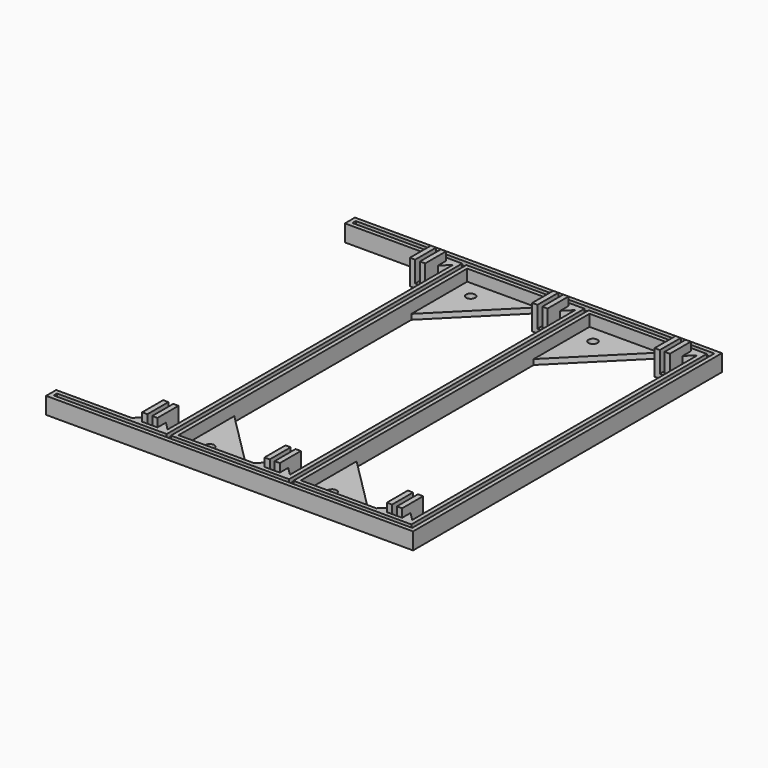
from build123d import *

# Parameters (mm, degrees)
F1_DEPTH     = 8
F2_W         = 2.5
F2_H         = 12.5
F3_DEPTH     = 4
F4_W         = 7.3
F4_H         = 12.5
F5_DEPTH     = 2
F7_DEPTH     = 2
F9_DEPTH     = 2
F10_T1_DEPTH = 8
F11_R        = 2.15
F12_DEPTH    = 2.5


# Not quite as in the source:
# - a fillet or chamfer that OpenCascade refuses, or shapes differently, is made with other operations: its cross-section is extruded or revolved along the edge and cut away or added


with BuildPart() as f1:
    # F0 (on Top) → F1 (new body)
    with BuildSketch(Plane.XY):
        Polygon((87.45, 92), (-87.45, 92), (-87.45, 86), (-46.45, 86), (-46.45, 73.5), (-43.95, 73.5), (-43.95, 86), (-41.65, 86), (-41.65, 73.5), (-39.15, 73.5), (-39.15, 86), (-35.15, 86), (-35.15, 0), (-35.15, -86), (-39.15, -86), (-39.15, -73.5), (-41.65, -73.5), (-41.65, -86), (-43.95, -86), (-43.95, -73.5), (-46.45, -73.5), (-46.45, -86), (-87.45, -86), (-87.45, -92), (87.45, -92), (87.45, 0), align=None)
        Polygon((-29.15, -86), (-29.15, 0), (-29.15, 86), (11.85, 86), (11.85, 73.5), (14.35, 73.5), (14.35, 86), (16.65, 86), (16.65, 73.5), (19.15, 73.5), (19.15, 86), (23.15, 86), (23.15, 0), (23.15, -86), (19.15, -86), (19.15, -73.5), (16.65, -73.5), (16.65, -86), (14.35, -86), (14.35, -73.5), (11.85, -73.5), (11.85, -86), align=None, mode=Mode.SUBTRACT)
        Polygon((29.15, -86), (29.15, 0), (29.15, 86), (70.15, 86), (70.15, 73.5), (72.65, 73.5), (72.65, 86), (74.95, 86), (74.95, 73.5), (77.45, 73.5), (77.45, 86), (81.45, 86), (81.45, 0), (81.45, -86), (77.45, -86), (77.45, -73.5), (74.95, -73.5), (74.95, -86), (72.65, -86), (72.65, -73.5), (70.15, -73.5), (70.15, -86), align=None, mode=Mode.SUBTRACT)
    extrude(amount=F1_DEPTH)

    # F2 (on face) → F3 (join)
    with BuildSketch(Plane.XY.offset(8)):
        with Locations((-40.4, 79.75)):
            Rectangle(F2_W, F2_H)
        with Locations((-45.2, 79.75)):
            Rectangle(F2_W, F2_H)
        with Locations((13.1, 79.75)):
            Rectangle(F2_W, F2_H)
        with Locations((17.9, 79.75)):
            Rectangle(F2_W, F2_H)
        with Locations((76.2, 79.75)):
            Rectangle(F2_W, F2_H)
        with Locations((71.4, 79.75)):
            Rectangle(F2_W, F2_H)
        with Locations((76.2, -79.75)):
            Rectangle(F2_W, F2_H)
        with Locations((71.4, -79.75)):
            Rectangle(F2_W, F2_H)
        with Locations((-40.4, -79.75)):
            Rectangle(F2_W, F2_H)
        with Locations((-45.2, -79.75)):
            Rectangle(F2_W, F2_H)
        with Locations((17.9, -79.75)):
            Rectangle(F2_W, F2_H)
        with Locations((13.1, -79.75)):
            Rectangle(F2_W, F2_H)
    extrude(amount=F3_DEPTH)

    # F4 (on face) → F5 (join)
    with BuildSketch(Plane(origin=(0, 0, 0), x_dir=(1, 0, 0), z_dir=(0, 0, -1))):
        with Locations((-42.8, 79.75)):
            Rectangle(F4_W, F4_H)
        with Locations((15.5, 79.75)):
            Rectangle(F4_W, F4_H)
        with Locations((73.8, 79.75)):
            Rectangle(F4_W, F4_H)
        with Locations((15.5, -79.75)):
            Rectangle(F4_W, F4_H)
        with Locations((-42.8, -79.75)):
            Rectangle(F4_W, F4_H)
        with Locations((73.8, -79.75)):
            Rectangle(F4_W, F4_H)
    extrude(amount=-F5_DEPTH)

    # F6 (on face) → F7 (cut)
    with BuildSketch(Plane.XY.offset(8)):
        Polygon((85.45, 90), (-85.45, 90), (-85.45, 88), (-33.15, 88), (-33.15, 0), (-33.15, -88), (-85.45, -88), (-85.45, -90), (85.45, -90), (85.45, 0), align=None)
        Polygon((25.15, 88), (25.15, 0), (25.15, -88), (-31.15, -88), (-31.15, 0), (-31.15, 88), align=None, mode=Mode.SUBTRACT)
        Polygon((27.15, 88), (83.45, 88), (83.45, 0), (83.45, -88), (27.15, -88), (27.15, 0), align=None, mode=Mode.SUBTRACT)
    extrude(amount=-F7_DEPTH, mode=Mode.SUBTRACT)

    # F8 (on face) → F9 (cut)
    with BuildSketch(Plane(origin=(0, 0, 0), x_dir=(1, 0, 0), z_dir=(0, 0, -1))):
        Polygon((85.45, 90), (-85.45, 90), (-85.45, 88), (-33.15, 88), (-33.15, 0), (-33.15, -88), (-85.45, -88), (-85.45, -90), (85.45, -90), (85.45, 0), align=None)
        Polygon((25.15, 88), (25.15, 0), (25.15, -88), (-31.15, -88), (-31.15, 0), (-31.15, 88), align=None, mode=Mode.SUBTRACT)
        Polygon((27.15, 88), (83.45, 88), (83.45, 0), (83.45, -88), (27.15, -88), (27.15, 0), align=None, mode=Mode.SUBTRACT)
    extrude(amount=-F9_DEPTH, mode=Mode.SUBTRACT)

    # F10: chamfer of 5 on 12 edges, made by hand

    # F10_s2 → F10_t1 (join)
    with BuildSketch(Plane.XY):
        Polygon((-39.15, 81), (-34.15, 86), (-39.15, 86), align=None)
        Polygon((-51.45, 86), (-46.45, 81), (-46.45, 86), align=None)
        Polygon((11.85, 81), (6.85, 86), (11.85, 86), align=None)
        Polygon((24.15, 86), (19.15, 81), (19.15, 86), align=None)
        Polygon((77.45, 81), (82.45, 86), (77.45, 86), align=None)
        Polygon((65.15, 86), (70.15, 81), (70.15, 86), align=None)
        Polygon((77.45, -81), (82.45, -86), (77.45, -86), align=None)
        Polygon((65.15, -86), (70.15, -81), (70.15, -86), align=None)
        Polygon((11.85, -81), (6.85, -86), (11.85, -86), align=None)
        Polygon((-51.45, -86), (-46.45, -81), (-46.45, -86), align=None)
        Polygon((-39.15, -81), (-34.15, -86), (-39.15, -86), align=None)
        Polygon((24.15, -86), (19.15, -81), (19.15, -86), align=None)
    extrude(amount=F10_T1_DEPTH)

    # F11 (on face) → F12 (join)
    with BuildSketch(Plane(origin=(0, 0, 0), x_dir=(1, 0, 0), z_dir=(0, 0, -1))):
        Polygon((29.15, -52.7659812842), (29.15, -86), (62.3840187158, -86), align=None)
        with Locations((37.4585046789, -77.6914953211)):
            Circle(F11_R, mode=Mode.SUBTRACT)
        Polygon((29.15, 86), (29.15, 52.7659812842), (62.3840187158, 86), align=None)
        with Locations((37.4585046789, 77.6914953211)):
            Circle(F11_R, mode=Mode.SUBTRACT)
        Polygon((-29.15, -52.7659812842), (-29.15, -86), (4.0840187158, -86), align=None)
        with Locations((-20.8414953211, -77.6914953211)):
            Circle(F11_R, mode=Mode.SUBTRACT)
        Polygon((-29.15, 86), (-29.15, 52.7659812842), (4.0840187158, 86), align=None)
        with Locations((-20.8414953211, 77.6914953211)):
            Circle(F11_R, mode=Mode.SUBTRACT)
    extrude(amount=-F12_DEPTH)


solid = f1.part
